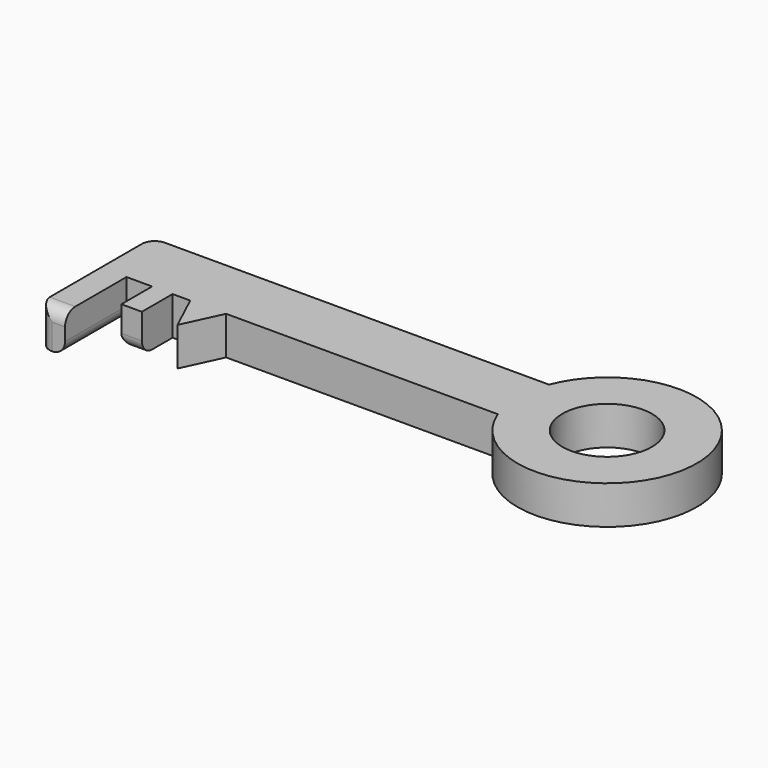
from build123d import *

# Parameters (mm, degrees)
F0_R     = 17.5
F0_W     = 10
F0_H     = 30
F0_W_2   = 8
F0_H_2   = 15
F1_DEPTH = 15
F2_R     = 4.99999


# Not quite as in the source:
# - a fillet or chamfer is up to 0.001 mm smaller than in the source, because OpenCascade refuses the exact size


with BuildPart() as f1:
    # F0 (on Top) → F1 (new body)
    with BuildSketch(Plane.XY):
        Polygon((-106.1073173197, 0), (0, 0), (0, 25), (-155, 25), (-155, 0), (-145, 0), (-135, 0), (-127, 0), (-120.1073173197, 0), align=None)
        with BuildLine():
            Line((0, 25), (0, 0))
            ThreePointArc((0, 0), (67.6917420766, 12.5), (0, 25))
        make_face()
        with Locations((32.6917420766, 12.5)):
            Circle(F0_R, mode=Mode.SUBTRACT)
        Polygon((-113.1073173197, -15), (-106.1073173197, 0), (-120.1073173197, 0), align=None)
        with Locations((-150, -15)):
            Rectangle(F0_W, F0_H)
        with Locations((-131, -7.5)):
            Rectangle(F0_W_2, F0_H_2)
    extrude(amount=F1_DEPTH)

    # F2 (radius 5 in the source; OpenCascade refuses exactly that, so slightly less here)
    f2_edges = [f1.edges().sort_by_distance(p)[0] for p in [
        (-155, 25, 7.5),
        (-155, -30, 7.5),
        (-150, -30, 15),
        (-145, -15, 0),
        (-140, 0, 0),
        (-135, -7.5, 0),
        (-131, -15, 0),
    ]]
    fillet(f2_edges, radius=F2_R)


solid = f1.part
